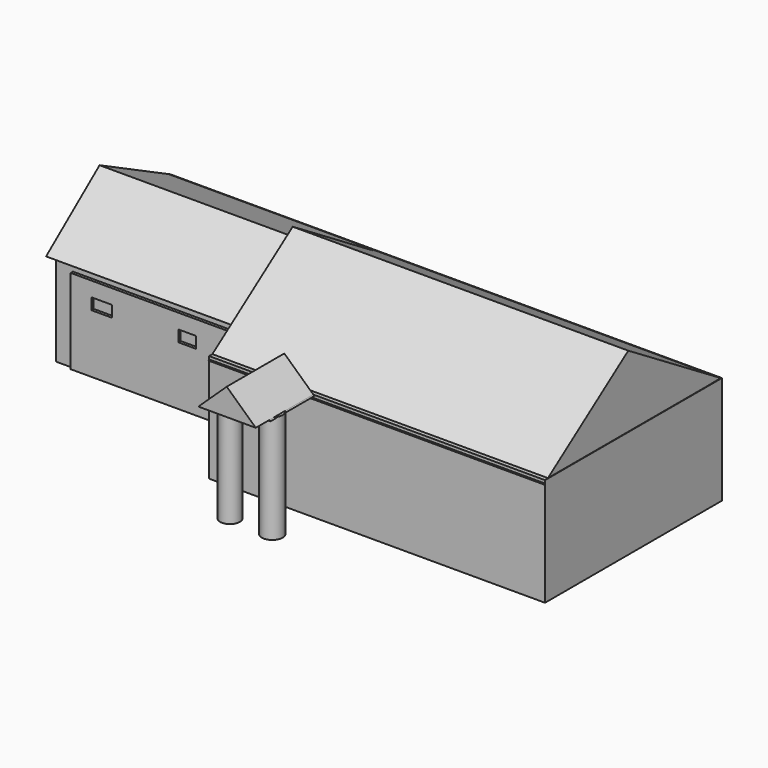
from build123d import *

# Parameters (mm, degrees)
F0_W      = 1.8879286945
F0_H      = 11.4653147757
F0_W_2    = 1.7881840467
F0_H_2    = 24.578695884
F0_W_3    = 13.0486488342
F0_H_3    = 2.4496505503
F1_DEPTH  = 38.1
F2_T      = -2.54
F3_R      = 3.6462481821
F4_DEPTH  = 38.1
F3_R_2    = 3.4707937143
F6_DEPTH  = 118.4148
F10_DEPTH = 76.3778
F11_W     = 55.7948499918
F11_H     = 29.9196355045
F11_W_2   = 7.285926491
F11_H_2   = 4.0264315903
F11_W_3   = 6.327252835
F12_DEPTH = 1.016
F14_DEPTH = 19.3802
F17_DEPTH = 25.4


# Not quite as in the source:
# - the program builds the solid bodies; features that only make, move or delete a surface that nothing else refers to are left out


with BuildPart() as f1:
    # F0 (on Top) → F1 (new body)
    with BuildSketch(Plane.XY):
        Polygon((115.5052706599, 46.1629368365), (0, 46.1629368365), (0, 36.2635403872), (5.0127906725, 33.348493278), (3.9305194266, 31.4873915519), (-2.1358516533, 33.348493278), (-2.1358516533, 46.1629368365), (-73.9798247814, 46.1629368365), (-73.9798247814, 2.8401890304), (-2.1358516533, 2.8401890304), (-2.1358516533, 25.5750287324), (0, 25.5750287324), (0, 0), (32.6135978103, 0), (32.6135978103, -10.8203999698), (36.2712033093, -12.9540003836), (34.8249944744, -15.4332187757), (30.5749002367, -12.9540003836), (30.5749002367, -1.6563893296), (2.5344253518, -1.6563893296), (2.5344253518, -27.0283464342), (30.5749002367, -27.0283464342), (30.5749002367, -18.0092640221), (32.6135978103, -18.0092640221), (32.6135978103, -27.0283464342), (48.8130263984, -27.0283464342), (48.8130263984, -15.5630316585), (50.7009550929, -15.5630316585), (50.7009550929, -27.0283464342), (79.7093436122, -27.0283464342), (79.7093436122, -2.4496505503), (50.7009550929, -2.4496505503), (50.7009550929, -7.0923493578), (52.741076349, -6.0931874175), (53.6812692881, -8.0129038543), (48.8130263984, -10.3971557692), (48.8130263984, 0), (93.6689444834, 0), (97.4417412263, -6.2941650698), (95.5842658877, -7.4075576849), (92.6124379039, -2.4496505503), (81.4975276589, -2.4496505503), (81.4975276589, -27.0283464342), (115.5052706599, -27.0283464342), (115.5052706599, -2.4496505503), (102.4566218257, -2.4496505503), (102.4566218257, 0), (115.5052706599, 0), align=None)
        Polygon((0, 46.1629368365), (0, 49.8348027468), (-76.5047967434, 49.8348027468), (-76.5047967434, 0), (0, 0), (0, 25.5750287324), (-2.1358516533, 25.5750287324), (-2.1358516533, 2.8401890304), (-73.9798247814, 2.8401890304), (-73.9798247814, 46.1629368365), (-2.1358516533, 46.1629368365), (-2.1358516533, 33.348493278), (3.9305194266, 31.4873915519), (5.0127906725, 33.348493278), (0, 36.2635403872), align=None)
        Polygon((32.6135978103, 0), (0, 0), (0, -28.1940009445), (32.6135978103, -28.1940009445), (32.6135978103, -27.0283464342), (32.6135978103, -18.0092640221), (30.5749002367, -18.0092640221), (30.5749002367, -27.0283464342), (2.5344253518, -27.0283464342), (2.5344253518, -1.6563893296), (30.5749002367, -1.6563893296), (30.5749002367, -12.9540003836), (34.8249944744, -15.4332187757), (36.2712033093, -12.9540003836), (32.6135978103, -10.8203999698), align=None)
        with Locations((49.7569907457, -21.2956890464)):
            Rectangle(F0_W, F0_H)
        Polygon((32.6135978103, -28.1940009445), (50.7009550929, -28.1940009445), (50.7009550929, -27.0283464342), (48.8130263984, -27.0283464342), (32.6135978103, -27.0283464342), align=None)
        Polygon((50.7009550929, -2.4496505503), (79.7093436122, -2.4496505503), (81.4975276589, -2.4496505503), (92.6124379039, -2.4496505503), (95.5842658877, -7.4075576849), (97.4417412263, -6.2941650698), (93.6689444834, 0), (48.8130263984, 0), (48.8130263984, -10.3971557692), (53.6812692881, -8.0129038543), (52.741076349, -6.0931874175), (50.7009550929, -7.0923493578), align=None)
        with Locations((80.6034356356, -14.7389984922)):
            Rectangle(F0_W_2, F0_H_2)
        Polygon((118.5672059655, 49.8348027468), (0, 49.8348027468), (0, 46.1629368365), (115.5052706599, 46.1629368365), (115.5052706599, 0), (115.5052706599, -2.4496505503), (115.5052706599, -27.0283464342), (81.4975276589, -27.0283464342), (79.7093436122, -27.0283464342), (50.7009550929, -27.0283464342), (50.7009550929, -28.1940009445), (118.5672059655, -28.1940009445), align=None)
        with Locations((108.9809462428, -1.2248252751)):
            Rectangle(F0_W_3, F0_H_3)
    extrude(amount=F1_DEPTH)

    # F2
    f2_openings = [f1.faces().sort_by_distance(p)[0] for p in [
        (30.819232, 14.934392, 38.1),
    ]]
    offset(amount=F2_T, openings=f2_openings, kind=Kind.INTERSECTION)

    # F5 (on Right) → F6 (join)
    with BuildSketch(Plane.YZ):
        Polygon((8.7074302137, 63.2784813643), (-28.5157766193, 36.8304103613), (49.4514331222, 38.2143817842), align=None)
    extrude(amount=F6_DEPTH)

    # F9 (on face) → F10 (join)
    with BuildSketch(Plane(origin=(0, 0, 0), x_dir=(0, -1, 0), z_dir=(-1, 0, 0))):
        Polygon((-18.9741293217, 53.3712290613), (-49.4514331222, 38.2143817842), (-2.54, 37.3816716864), (-2.54, 38.1), (0, 38.1), (0, 34.9335108109), (4.6135843263, 34.6274210994), align=None)
    extrude(amount=F10_DEPTH)

    # F11 (on face) → F12 (join)
    with BuildSketch(Plane.XZ):
        with Locations((-42.6739454269, 14.9598177522)):
            Rectangle(F11_W, F11_H)
        with Locations((-59.6424844116, 22.7295774966)):
            Rectangle(F11_W_2, F11_H_2, mode=Mode.SUBTRACT)
        with Locations((-29.444238171, 22.7295774966)):
            Rectangle(F11_W_3, F11_H_2, mode=Mode.SUBTRACT)
    extrude(amount=F12_DEPTH)


with BuildPart() as f4:
    # F3 (on Top) → F4 (new body)
    with BuildSketch(Plane.XY):
        with Locations((34.1883972287, -43.0675931275)):
            Circle(F3_R)
    extrude(amount=F4_DEPTH)


with BuildPart() as f4b:
    # F3 (on Top) → F4, piece 2 (new body)
    with BuildSketch(Plane.XY):
        with Locations((19.2820988595, -43.0675931275)):
            Circle(F3_R_2)
    extrude(amount=F4_DEPTH)


with BuildPart() as f14:
    # F13 (on face) → F14 (new body)
    with BuildSketch(Plane.XZ.offset(28.1940009445)):
        Polygon((26.5588965267, 47.5474819541), (16.544852101, 38.1), (36.8077256615, 38.1), align=None)
        Polygon((16.544852101, 38.1), (16.1166600883, 37.6960337162), (37.1683239937, 37.7675965428), (36.8077256615, 38.1), align=None)
    extrude(amount=F14_DEPTH)


with BuildPart() as f17:
    # F13 (on face) → F17 (new body)
    with BuildSketch(Plane.XZ.offset(28.1940009445)):
        Polygon((26.5588965267, 47.5474819541), (16.544852101, 38.1), (36.8077256615, 38.1), align=None)
    extrude(amount=F17_DEPTH)


solid = Compound([f1.part, f4.part, f4b.part, f14.part, f17.part])
